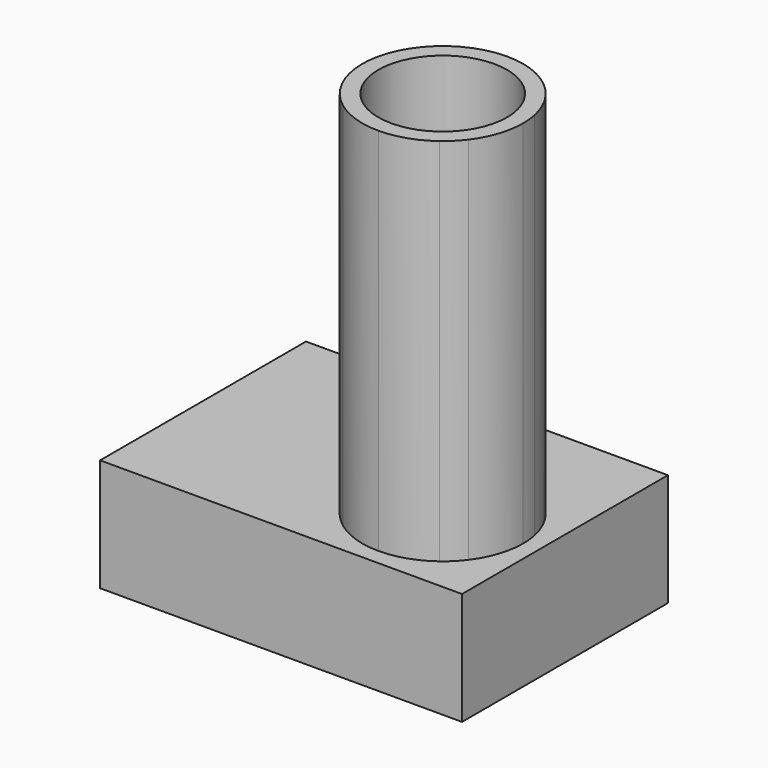
from build123d import *

# Parameters (mm, degrees)
F1_DEPTH = 14
F2_DEPTH = 60


with BuildPart() as f1:
    # F0 (on Top) → F1 (new body)
    with BuildSketch(Plane.XY):
        Polygon((0, 14), (0, 0), (45, 0), (45, 14), (43, 14), (43, 12), (43, 2), (33, 2), (2, 2), (2, 4), (2, 12), (2, 14), align=None)
        Polygon((0, 32), (0, 14), (2, 14), (2, 30), (33, 30), (41, 30), (43, 30), (43, 14), (45, 14), (45, 32), align=None)
        with BuildLine():
            Line((23.2020410745, 14), (2, 14))
            Line((2, 14), (2, 12))
            Line((2, 12), (23.0000000447, 12))
            ThreePointArc((23.0000000447, 12), (23.0506385149, 13.0050896201), (23.2020410745, 14))
        make_face()
        with BuildLine():
            Line((2, 30), (2, 14))
            Line((2, 14), (23.2020410745, 14))
            ThreePointArc((23.2020410745, 14), (26.6754447115, 19.7459666607), (33, 21.9999999553))
            Line((33, 21.9999999553), (33, 30))
            Line((33, 30), (2, 30))
        make_face()
        with BuildLine():
            Line((42.7979589255, 14), (43, 14))
            Line((43, 14), (43, 30))
            Line((43, 30), (41, 30))
            Line((41, 30), (41, 17.9999999255))
            ThreePointArc((41, 17.9999999255), (42.1209558342, 16.0997760642), (42.7979589255, 14))
        make_face()
        with BuildLine():
            Line((43, 12), (43, 14))
            Line((43, 14), (42.7979589255, 14))
            ThreePointArc((42.7979589255, 14), (42.9493614851, 13.0050896201), (42.9999999553, 12))
        make_face()
        with BuildLine():
            Line((23.0000000447, 12), (2, 12))
            Line((2, 12), (2, 4))
            Line((2, 4), (27.0000000745, 4))
            ThreePointArc((27.0000000745, 4), (24.0557281433, 7.5278640383), (23.0000000447, 12))
        make_face()
        with BuildLine():
            Line((25.2540333076, 14), (23.2020410745, 14))
            ThreePointArc((23.2020410745, 14), (23.0506385149, 13.0050896201), (23.0000000447, 12))
            Line((23.0000000447, 12), (25, 12))
            ThreePointArc((25, 12), (25.0637624299, 13.0080343399), (25.2540333076, 14))
        make_face()
        with BuildLine():
            ThreePointArc((33, 21.9999999553), (26.6754447115, 19.7459666607), (23.2020410745, 14))
            Line((23.2020410745, 14), (25.2540333076, 14))
            ThreePointArc((25.2540333076, 14), (28.1010205144, 18.3245553203), (33, 20))
            Line((33, 20), (33, 21.9999999553))
        make_face()
        with BuildLine():
            ThreePointArc((41, 6.0000000745), (42.4868329475, 8.8377223822), (42.9999999553, 12))
            ThreePointArc((42.9999999553, 12), (42.9493614851, 13.0050896201), (42.7979589255, 14))
            Line((42.7979589255, 14), (41, 14))
            Line((41, 14), (41, 12))
            Line((41, 12), (41, 6.0000000745))
        make_face()
        with BuildLine():
            Line((43, 2), (43, 12))
            ThreePointArc((42.9999999553, 12), (42.4868329475, 8.8377223822), (41, 6.0000000745))
            Line((41, 6.0000000745), (41, 4))
            Line((41, 4), (38.9999999255, 4))
            ThreePointArc((38.9999999255, 4), (36.1622776178, 2.5131670525), (33, 2.0000000447))
            Line((33, 2), (43, 2))
        make_face()
        with BuildLine():
            Line((41, 14), (42.7979589255, 14))
            ThreePointArc((42.7979589255, 14), (42.1209558342, 16.0997760642), (41, 17.9999999255))
            Line((41, 17.9999999255), (41, 14))
        make_face()
        with BuildLine():
            Line((27.0000000745, 4), (2, 4))
            Line((2, 4), (2, 2))
            Line((2, 2), (33, 2))
            ThreePointArc((33, 2.0000000447), (29.8377223822, 2.5131670525), (27.0000000745, 4))
        make_face()
        with BuildLine():
            Line((25, 12), (23.0000000447, 12))
            ThreePointArc((23.0000000447, 12), (24.0557281433, 7.5278640383), (27.0000000745, 4))
            Line((27.0000000745, 4), (33, 4))
            ThreePointArc((33, 4), (27.3431457505, 6.3431457505), (25, 12))
        make_face()
        with BuildLine():
            Line((41, 30), (33, 30))
            Line((33, 30), (33, 21.9999999553))
            ThreePointArc((33, 21.9999999553), (37.4721359617, 20.9442718567), (41, 17.9999999255))
            Line((41, 17.9999999255), (41, 30))
        make_face()
        with BuildLine():
            ThreePointArc((38.9999999255, 4), (40.0710677803, 4.9289322197), (41, 6.0000000745))
            Line((41, 6.0000000745), (41, 12))
            ThreePointArc((41, 12), (38.6568542495, 6.3431457505), (33, 4))
            Line((33, 4), (38.9999999255, 4))
        make_face()
        with BuildLine():
            Line((41, 4), (41, 6.0000000745))
            ThreePointArc((41, 6.0000000745), (40.0710677803, 4.9289322197), (38.9999999255, 4))
            Line((38.9999999255, 4), (41, 4))
        make_face()
        with BuildLine():
            Line((41, 12), (41, 14))
            Line((41, 14), (40.7459666924, 14))
            ThreePointArc((40.7459666924, 14), (40.9362375701, 13.0080343399), (41, 12))
        make_face()
        with BuildLine():
            Line((33, 4), (27.0000000745, 4))
            ThreePointArc((27.0000000745, 4), (29.8377223822, 2.5131670525), (33, 2.0000000447))
            ThreePointArc((33, 2.0000000447), (36.1622776178, 2.5131670525), (38.9999999255, 4))
            Line((38.9999999255, 4), (33, 4))
        make_face()
    extrude(amount=F1_DEPTH)

    # F0 (on Top) → F2 (join)
    with BuildSketch(Plane.XY):
        with BuildLine():
            Line((25.2540333076, 14), (23.2020410745, 14))
            ThreePointArc((23.2020410745, 14), (23.0506385149, 13.0050896201), (23.0000000447, 12))
            Line((23.0000000447, 12), (25, 12))
            ThreePointArc((25, 12), (25.0637624299, 13.0080343399), (25.2540333076, 14))
        make_face()
        with BuildLine():
            ThreePointArc((33, 21.9999999553), (26.6754447115, 19.7459666607), (23.2020410745, 14))
            Line((23.2020410745, 14), (25.2540333076, 14))
            ThreePointArc((25.2540333076, 14), (28.1010205144, 18.3245553203), (33, 20))
            Line((33, 20), (33, 21.9999999553))
        make_face()
        with BuildLine():
            ThreePointArc((41, 6.0000000745), (42.4868329475, 8.8377223822), (42.9999999553, 12))
            ThreePointArc((42.9999999553, 12), (42.9493614851, 13.0050896201), (42.7979589255, 14))
            Line((42.7979589255, 14), (41, 14))
            Line((41, 14), (41, 12))
            Line((41, 12), (41, 6.0000000745))
        make_face()
        with BuildLine():
            Line((41, 14), (42.7979589255, 14))
            ThreePointArc((42.7979589255, 14), (42.1209558342, 16.0997760642), (41, 17.9999999255))
            Line((41, 17.9999999255), (41, 14))
        make_face()
        with BuildLine():
            Line((25, 12), (23.0000000447, 12))
            ThreePointArc((23.0000000447, 12), (24.0557281433, 7.5278640383), (27.0000000745, 4))
            Line((27.0000000745, 4), (33, 4))
            ThreePointArc((33, 4), (27.3431457505, 6.3431457505), (25, 12))
        make_face()
        with BuildLine():
            ThreePointArc((41, 17.9999999255), (37.4721359617, 20.9442718567), (33, 21.9999999553))
            Line((33, 21.9999999553), (33, 20))
            ThreePointArc((33, 20), (37.8989794856, 18.3245553203), (40.7459666924, 14))
            Line((40.7459666924, 14), (41, 14))
            Line((41, 14), (41, 17.9999999255))
        make_face()
        with BuildLine():
            ThreePointArc((38.9999999255, 4), (40.0710677803, 4.9289322197), (41, 6.0000000745))
            Line((41, 6.0000000745), (41, 12))
            ThreePointArc((41, 12), (38.6568542495, 6.3431457505), (33, 4))
            Line((33, 4), (38.9999999255, 4))
        make_face()
        with BuildLine():
            Line((41, 12), (41, 14))
            Line((41, 14), (40.7459666924, 14))
            ThreePointArc((40.7459666924, 14), (40.9362375701, 13.0080343399), (41, 12))
        make_face()
        with BuildLine():
            Line((33, 4), (27.0000000745, 4))
            ThreePointArc((27.0000000745, 4), (29.8377223822, 2.5131670525), (33, 2.0000000447))
            ThreePointArc((33, 2.0000000447), (36.1622776178, 2.5131670525), (38.9999999255, 4))
            Line((38.9999999255, 4), (33, 4))
        make_face()
    extrude(amount=F2_DEPTH)


solid = f1.part
